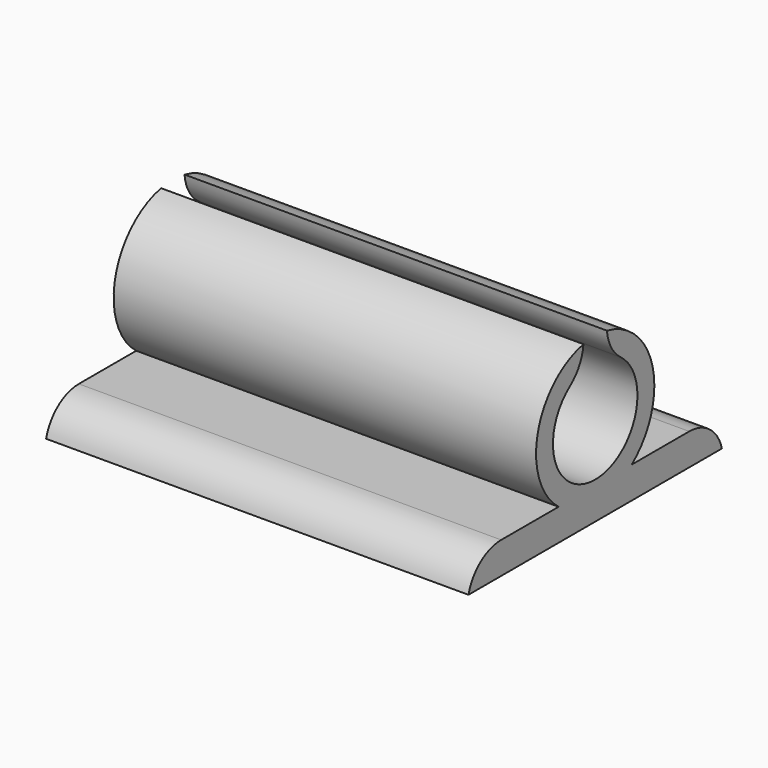
from build123d import *

# Parameters (mm, degrees)
F0_W        = 25.4
F0_H        = 19.05
F1_DEPTH    = 1.905
F3_DEPTH    = 12.7
F4_T1_DEPTH = 37.6967221242
F4_T3_DEPTH = 31.9335157919


# Not quite as in the source:
# - a fillet or chamfer that OpenCascade refuses, or shapes differently, is made with other operations: its cross-section is extruded or revolved along the edge and cut away or added


with BuildPart() as f1:
    # F0 (on Top) → F1 (new body)
    with BuildSketch(Plane.XY):
        Rectangle(F0_W, F0_H)
    extrude(amount=F1_DEPTH)

    # F2 (on Right) → F3 (join, symmetric)
    with BuildSketch(Plane.YZ):
        with BuildLine():
            ThreePointArc((-0.8833862371, 9.7538348994), (-4.3244369874, 6.4257362287), (-2.749630657, 1.905))
            Line((-2.749630657, 1.905), (2.749630657, 1.905))
            ThreePointArc((2.749630657, 1.905), (3.9987581366, 3.4563770351), (4.445, 5.3975))
            ThreePointArc((4.445, 5.3975), (3.4412698836, 8.2109829994), (0.8833862371, 9.7538348994))
            Line((0.8833862371, 9.7538348994), (0.8833862371, 8.4471317411))
            ThreePointArc((0.8833862371, 8.4471317411), (2.5382450929, 7.3048376336), (3.175, 5.3975))
            ThreePointArc((3.175, 5.3975), (-1.9073376336, 2.8592549071), (-0.8833862371, 8.4471317411))
            Line((-0.8833862371, 8.4471317411), (-0.8833862371, 9.7538348994))
        make_face()
    extrude(amount=F3_DEPTH, both=True)

    # F4: fillet of radius 2.54 on 4 edges, made by hand

    # F4_s2 → F4_t1 (cut)
    with BuildSketch(Plane.YZ.offset(-18.8483610621)):
        with BuildLine():
            ThreePointArc((-9.525, 0), (-8.6210815618, 1.3730463142), (-7.0656555752, 1.905))
            Line((-7.0656555752, 1.905), (-9.525, 1.905))
            Line((-9.525, 1.905), (-9.525, 0))
        make_face()
        with BuildLine():
            ThreePointArc((9.525, 0), (8.6210815618, 1.3730463142), (7.0656555752, 1.905))
            Line((7.0656555752, 1.905), (9.525, 1.905))
            Line((9.525, 1.905), (9.525, 0))
        make_face()
    extrude(amount=F4_T1_DEPTH, mode=Mode.SUBTRACT)

    # F4_s4 → F4_t3 (cut)
    with BuildSketch(Plane.YZ.offset(-15.9667578959)):
        with BuildLine():
            ThreePointArc((0.8833862371, 9.7538348994), (1.1966765002, 8.7408723938), (1.8962102849, 7.9440685845))
            ThreePointArc((1.8962102849, 7.9440685845), (1.4123764871, 8.2410572192), (0.8833862371, 8.4471317411))
            Line((0.8833862371, 8.4471317411), (0.8833862371, 9.7538348994))
        make_face()
        with BuildLine():
            ThreePointArc((-1.8962102849, 7.9440685845), (-1.1966765002, 8.7408723938), (-0.8833862371, 9.7538348994))
            Line((-0.8833862371, 9.7538348994), (-0.8833862371, 8.4471317411))
            ThreePointArc((-0.8833862371, 8.4471317411), (-1.4123764871, 8.2410572192), (-1.8962102849, 7.9440685845))
        make_face()
    extrude(amount=F4_T3_DEPTH, mode=Mode.SUBTRACT)


solid = f1.part
